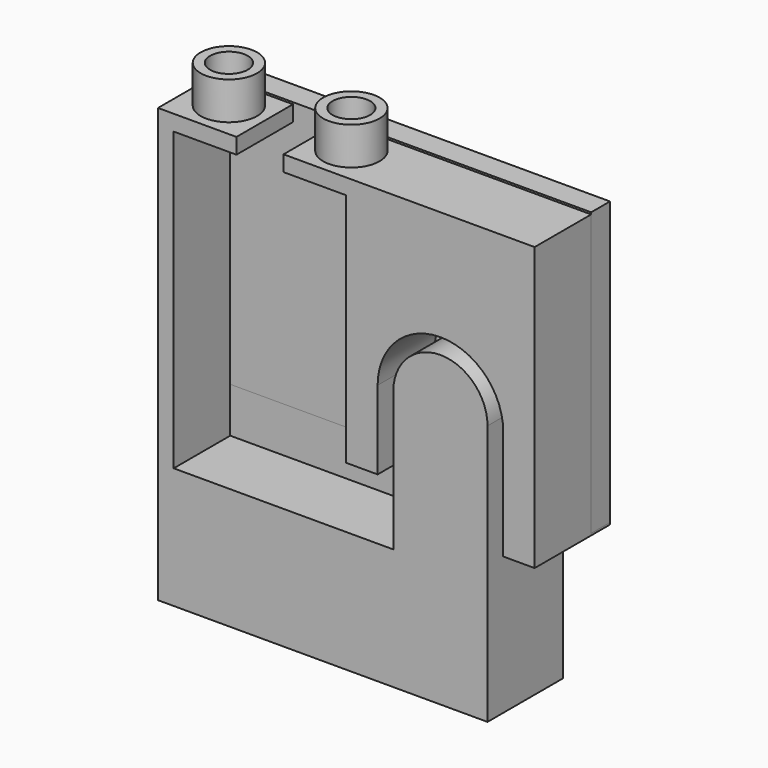
from build123d import *

# Parameters (mm, degrees)
F1_DEPTH  = 15.875
F0_W      = 2.6458333332
F0_H      = 42.3358732487
F2_W      = 63.5
F2_H      = 47.625
F2_R      = 3.175
F3_DEPTH  = 3.96875
F4_DEPTH  = 6.35
F5_R      = 4.7625
F5_R_2    = 3.175
F6_DEPTH  = 6.35
F7_R      = 3.175
F8_DEPTH  = 25.4
F9_W      = 55.5296598673
F9_H      = 15.875
F10_DEPTH = 25.4
F11_W     = 37.0088265341
F11_H     = 15.875
F12_DEPTH = 7.62
F13_W     = 37.0088265341
F13_H     = 3.96875
F14_DEPTH = 25.4


# Not quite as in the source:
# - a feature names something its author has since deleted; it is built from what else it names


with BuildPart() as f1:
    # F0 (on Front) → F1 (new body)
    with BuildSketch(Plane.XZ):
        with BuildLine():
            Line((0, 44.979166582), (-31.75, 44.979166582))
            Line((-31.75, 44.979166582), (-31.75, 42.3358732487))
            Line((-31.75, 42.3358732487), (-31.75, 2.6458333332))
            Line((-31.75, 2.6458333332), (-26.4583333333, 2.6458333332))
            Line((-26.4583333333, 2.6458333332), (-26.4583333333, 15.875))
            ThreePointArc((-26.4583333333, 15.875), (-15.875, 26.4583333333), (-5.2916666667, 15.875))
            Line((-5.2916666667, 15.875), (-5.2916666667, 0))
            Line((-5.2916666667, 0), (0, 0))
            Line((0, 0), (0, 44.979166582))
        make_face()
        Polygon((0, -2.6458333333), (0, 0), (-5.2916666667, 0), (-5.309548229, 0), (-5.309548229, -2.6458333333), align=None)
        Polygon((-31.75, 42.3358732487), (-31.75, 44.979166582), (-34.3958333316, 44.979166582), (-37.0416664956, 44.979166582), (-42.3110765377, 44.979166582), (-42.3110765377, 42.3358732487), (-37.0416664956, 42.3358732487), (-34.3958333316, 42.3358732487), align=None)
    extrude(amount=F1_DEPTH)


with BuildPart() as f1b:
    # F0 (on Front) → F1, piece 2 (new body)
    with BuildSketch(Plane.XZ):
        with BuildLine():
            Line((-23.8125, 0), (-7.9375, 0))
            Line((-7.9375, 0), (-7.9375, 15.875))
            ThreePointArc((-7.9375, 15.875), (-15.875, 23.8125), (-23.8125, 15.875))
            Line((-23.8125, 15.875), (-23.8125, 0))
        make_face()
        Polygon((-26.4583333333, 0), (-31.75, 0), (-60.8213265341, 0), (-63.4671598673, 0), (-63.4671598673, -2.6458333333), (-7.9375, -2.6458333333), (-7.9375, 0), (-23.8125, 0), align=None)
        with Locations((-62.1442432007, 21.1679366243)):
            Rectangle(F0_W, F0_H)
        Polygon((-50.2485765377, 42.3358732487), (-50.2485765377, 44.979166582), (-55.5296598693, 44.979166582), (-58.175493201, 44.979166582), (-63.4671598673, 44.979166582), (-63.4671598673, 42.3358732487), (-60.8213265341, 42.3358732487), (-58.175493201, 42.3358732487), (-55.5296598693, 42.3358732487), align=None)
    extrude(amount=F1_DEPTH)


with BuildPart() as f3:
    # F2 (on Front) → F3 (new body)
    with BuildSketch(Plane.XZ):
        with Locations((-31.75, 21.4839725468)):
            Rectangle(F2_W, F2_H)
        with Locations((-53.975, 7.1964725468)):
            Circle(F2_R, mode=Mode.SUBTRACT)
        with Locations((-9.525, 7.1964725468)):
            Circle(F2_R, mode=Mode.SUBTRACT)
        with Locations((-52.284011212, 35.7714725468)):
            Circle(F2_R, mode=Mode.SUBTRACT)
        with Locations((-9.525, 35.7714725468)):
            Circle(F2_R, mode=Mode.SUBTRACT)
        with Locations((-52.284011212, 35.7714725468)):
            Circle(F2_R)
        with Locations((-53.975, 7.1964725468)):
            Circle(F2_R)
        with Locations((-9.525, 7.1964725468)):
            Circle(F2_R)
        with Locations((-9.525, 35.7714725468)):
            Circle(F2_R)
    extrude(amount=F3_DEPTH)


with BuildPart() as f4:
    # F2 (on Front) → F4 (new body)
    with BuildSketch(Plane.XZ):
        with Locations((-9.525, 35.7714725468)):
            Circle(F2_R)
    extrude(amount=-F4_DEPTH)


with BuildPart() as f4b:
    # F2 (on Front) → F4, piece 2 (new body)
    with BuildSketch(Plane.XZ):
        with Locations((-52.284011212, 35.7714725468)):
            Circle(F2_R)
    extrude(amount=-F4_DEPTH)


with BuildPart() as f4c:
    # F2 (on Front) → F4, piece 3 (new body)
    with BuildSketch(Plane.XZ):
        with Locations((-9.525, 7.1964725468)):
            Circle(F2_R)
    extrude(amount=-F4_DEPTH)


with BuildPart() as f4d:
    # F2 (on Front) → F4, piece 4 (new body)
    with BuildSketch(Plane.XZ):
        with Locations((-53.975, 7.1964725468)):
            Circle(F2_R)
    extrude(amount=-F4_DEPTH)


with BuildPart() as f6:
    # F5 (on face) → F6 (new body)
    with BuildSketch(Plane.XY.offset(44.979166582)):
        with Locations((-56.5985765377, -9.525)):
            Circle(F5_R)
        with Locations((-56.5985765377, -9.525)):
            Circle(F5_R_2, mode=Mode.SUBTRACT)
    extrude(amount=F6_DEPTH)


with BuildPart() as f6b:
    # F5 (on face) → F6, piece 2 (new body)
    with BuildSketch(Plane.XY.offset(44.979166582)):
        with Locations((-35.9610765377, -9.525)):
            Circle(F5_R)
        with Locations((-35.9610765377, -9.525)):
            Circle(F5_R_2, mode=Mode.SUBTRACT)
    extrude(amount=F6_DEPTH)


with BuildPart() as f8_tool:
    # F7 (on face) → F8 (new body)
    with BuildSketch(Plane.XY.offset(44.979166582)):
        with Locations((-35.9610765377, -9.525)):
            Circle(F7_R)
        with Locations((-56.5985765377, -9.525)):
            Circle(F7_R)
    extrude(amount=-F8_DEPTH)


with BuildPart() as f1_1:
    add(f1.part)

    # F8: cut by f8_tool
    add(f8_tool.part, mode=Mode.SUBTRACT)


with BuildPart() as f1b_1:
    add(f1b.part)

    # F8: cut by f8_tool
    add(f8_tool.part, mode=Mode.SUBTRACT)

    # F9 (on face) → F10 (join)
    with BuildSketch(Plane(origin=(0, 0, -2.6458333333), x_dir=(1, 0, 0), z_dir=(0, 0, -1))):
        with Locations((-35.7023299336, 7.9375)):
            Rectangle(F9_W, F9_H)
    extrude(amount=F10_DEPTH)


with BuildPart() as f12_tool:
    # F11 (on face) → F12 (new body)
    with BuildSketch(Plane.XY):
        with Locations((-42.3169132671, -7.9375)):
            Rectangle(F11_W, F11_H)
    extrude(amount=-F12_DEPTH)


with BuildPart() as f1b_2:
    add(f1b_1.part)

    # F12: cut by f12_tool
    add(f12_tool.part, mode=Mode.SUBTRACT)


with BuildPart() as f3_1:
    add(f3.part)

    # F12: cut by f12_tool
    add(f12_tool.part, mode=Mode.SUBTRACT)


with BuildPart() as f14:
    # F13 (on face) → F14 (new body)
    with BuildSketch(Plane(origin=(0, 0, 0), x_dir=(1, 0, 0), z_dir=(0, 0, -1))):
        with Locations((-42.3169132671, 1.984375)):
            Rectangle(F13_W, F13_H)
    extrude(amount=F14_DEPTH)


solid = Compound([f4.part, f4b.part, f4c.part, f4d.part, f6.part, f6b.part, f1_1.part, f1b_2.part, f3_1.part, f14.part])
